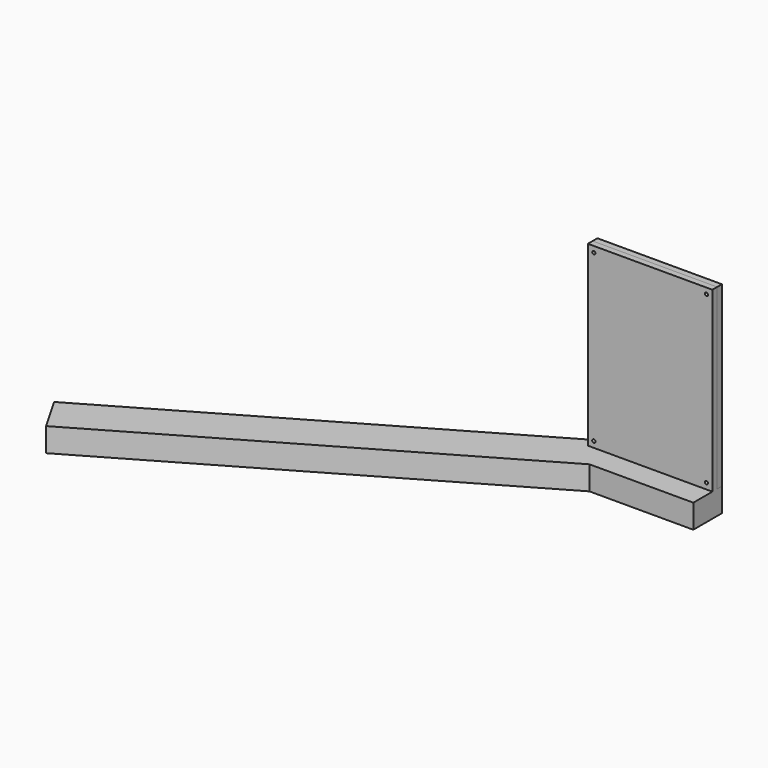
from build123d import *

# Parameters (mm, degrees)
F0_W      = 265.2573054
F0_H      = 378.7020874
F1_DEPTH  = 12.7
F2_DEPTH  = 3.302
F3_W      = 76.2
F3_H      = 50.8
F3_W_2    = 69.85
F3_H_2    = 44.45
F4_DEPTH  = 265.2573054
F6_DEPTH  = 50.8
F7_DEPTH  = 914.4
F8_W      = 265.2573054
F8_H      = 378.7020874
F8_R      = 3.4544
F9_DEPTH  = 12.7
F11_W     = 76.2
F11_H     = 50.8
F12_DEPTH = 3.175


with BuildPart() as f1:
    # F0 (on Front) → F1 (new body)
    with BuildSketch(Plane.XZ):
        with Locations((148.0387565, -1.27e-05)):
            Rectangle(F0_W, F0_H)
        with BuildLine():
            ThreePointArc((24.6557038, -176.6510564), (28.1101038, -173.1966564), (31.5645038, -176.6510564))
            ThreePointArc((31.5645038, -176.6510564), (28.1101038, -180.1054564), (24.6557038, -176.6510564))
        make_face(mode=Mode.SUBTRACT)
        with BuildLine():
            ThreePointArc((264.5130092, -176.6510564), (267.9674092, -173.1966564), (271.4218092, -176.6510564))
            ThreePointArc((271.4218092, -176.6510564), (267.9674092, -180.1054564), (264.5130092, -176.6510564))
        make_face(mode=Mode.SUBTRACT)
        with BuildLine():
            ThreePointArc((24.6557038, 176.651031), (28.1101038, 180.105431), (31.5645038, 176.651031))
            ThreePointArc((31.5645038, 176.651031), (28.1101038, 173.196631), (24.6557038, 176.651031))
        make_face(mode=Mode.SUBTRACT)
        with BuildLine():
            ThreePointArc((264.5130092, 176.651031), (267.9674092, 180.105431), (271.4218092, 176.651031))
            ThreePointArc((271.4218092, 176.651031), (267.9674092, 173.196631), (264.5130092, 176.651031))
        make_face(mode=Mode.SUBTRACT)
    extrude(amount=F1_DEPTH)


with BuildPart() as f1b:
    # F0 (on Front) → F1, piece 2 (new body)
    with BuildSketch(Plane.XZ):
        with BuildLine():
            Line((-259.816473, -139.4988066), (-259.809869, 139.9750058))
            ThreePointArc((-259.8098689962, 139.9750058), (-255.6250403922, 150.0775804789), (-245.522369, 154.2621756))
            Line((-245.522369, 154.2621756), (-50.5753624, 154.2621756))
            ThreePointArc((-50.5753624, 154.2621756), (-40.4724665013, 150.0773559726), (-36.2878624033, 139.9743708))
            Line((-36.2878624, 139.9743708), (-36.2944664, -139.4994416))
            ThreePointArc((-36.2944664038, -139.4994416), (-40.4792950078, -149.6020162789), (-50.5819664, -153.7866114))
            Line((-50.5819664, -153.7866114), (-132.307457, -153.7866114))
            ThreePointArc((-132.307457, -153.7866114), (-134.4627184691, -154.6793499309), (-135.355457, -156.8346114))
            Line((-135.355457, -156.8346114), (-135.355457, -171.7670174))
            Line((-135.355457, -171.7670174), (-135.355457, -187.919233))
            Line((-135.355457, -187.919233), (-135.355457, -189.3510564))
            Line((-135.355457, -189.3510564), (-15.4101038, -189.3510564))
            Line((-15.4101038, -189.3510564), (-15.4101038, 189.351031))
            Line((-15.4101038, 189.351031), (-280.6674092, 189.351031))
            Line((-280.6674092, 189.351031), (-280.6674092, -189.3510564))
            Line((-280.6674092, -189.3510564), (-160.755457, -189.3510564))
            Line((-160.755457, -189.3510564), (-160.755457, -187.919233))
            Line((-160.755457, -187.919233), (-160.755457, -171.7670174))
            Line((-160.755457, -171.7670174), (-160.755457, -156.8346114))
            ThreePointArc((-160.755457, -156.8346114), (-161.6481955309, -154.6793499309), (-163.803457, -153.7866114))
            Line((-163.803457, -153.7866114), (-245.528973, -153.7866114))
            ThreePointArc((-245.528973, -153.7866114), (-255.6318688987, -149.6017917726), (-259.8164729967, -139.4988066))
        make_face()
        with BuildLine():
            ThreePointArc((-271.4218092, -176.6510564), (-267.9674092, -173.1966564), (-264.5130092, -176.6510564))
            ThreePointArc((-264.5130092, -176.6510564), (-267.9674092, -180.1054564), (-271.4218092, -176.6510564))
        make_face(mode=Mode.SUBTRACT)
        with BuildLine():
            ThreePointArc((-31.5645038, -176.6510564), (-28.1101038, -173.1966564), (-24.6557038, -176.6510564))
            ThreePointArc((-24.6557038, -176.6510564), (-28.1101038, -180.1054564), (-31.5645038, -176.6510564))
        make_face(mode=Mode.SUBTRACT)
        with BuildLine():
            ThreePointArc((-271.4218092, 176.651031), (-267.9674092, 180.105431), (-264.5130092, 176.651031))
            ThreePointArc((-264.5130092, 176.651031), (-267.9674092, 173.196631), (-271.4218092, 176.651031))
        make_face(mode=Mode.SUBTRACT)
        with BuildLine():
            ThreePointArc((-31.5645038, 176.651031), (-28.1101038, 180.105431), (-24.6557038, 176.651031))
            ThreePointArc((-24.6557038, 176.651031), (-28.1101038, 173.196631), (-31.5645038, 176.651031))
        make_face(mode=Mode.SUBTRACT)
    extrude(amount=F1_DEPTH)

    # F0 (on Front) → F2 (join)
    with BuildSketch(Plane.XZ):
        with BuildLine():
            ThreePointArc((-245.522369, 154.2621756), (-255.6250403922, 150.0775804789), (-259.8098689962, 139.9750058))
            Line((-259.809869, 139.9750058), (-259.816473, -139.4988066))
            ThreePointArc((-259.8164729967, -139.4988066), (-255.6318688987, -149.6017917726), (-245.528973, -153.7866114))
            Line((-245.528973, -153.7866114), (-163.803457, -153.7866114))
            ThreePointArc((-163.803457, -153.7866114), (-161.6481955309, -154.6793499309), (-160.755457, -156.8346114))
            Line((-160.755457, -156.8346114), (-160.755457, -171.7670174))
            Line((-160.755457, -171.7670174), (-160.755457, -187.919233))
            Line((-160.755457, -187.919233), (-160.755457, -189.3510564))
            Line((-160.755457, -189.3510564), (-135.355457, -189.3510564))
            Line((-135.355457, -189.3510564), (-135.355457, -187.919233))
            Line((-135.355457, -187.919233), (-135.355457, -171.7670174))
            Line((-135.355457, -171.7670174), (-135.355457, -156.8346114))
            ThreePointArc((-135.355457, -156.8346114), (-134.4627184691, -154.6793499309), (-132.307457, -153.7866114))
            Line((-132.307457, -153.7866114), (-50.5819664, -153.7866114))
            ThreePointArc((-50.5819664, -153.7866114), (-40.4792950078, -149.6020162789), (-36.2944664038, -139.4994416))
            Line((-36.2944664, -139.4994416), (-36.2878624, 139.9743708))
            ThreePointArc((-36.2878624033, 139.9743708), (-40.4724665013, 150.0773559726), (-50.5753624, 154.2621756))
            Line((-50.5753624, 154.2621756), (-245.522369, 154.2621756))
        make_face()
        with BuildLine():
            ThreePointArc((-241.6466592, -129.499233), (-243.8917232303, -128.5692970303), (-244.8216592, -126.324233))
            Line((-244.8216592, -126.324233), (-244.8216592, 126.324741))
            ThreePointArc((-244.8216592, 126.324741), (-243.8917232303, 128.5698050303), (-241.6466592, 129.499741))
            Line((-241.6466592, 129.499741), (-54.6371526, 129.499741))
            ThreePointArc((-54.6371526, 129.499741), (-52.3920885697, 128.5698050303), (-51.4621526, 126.324741))
            Line((-51.4621526, 126.324741), (-51.4621526, -126.324233))
            ThreePointArc((-51.4621526, -126.324233), (-52.3920885697, -128.5692970303), (-54.6371526, -129.499233))
            Line((-54.6371526, -129.499233), (-241.6466592, -129.499233))
        make_face(mode=Mode.SUBTRACT)
        with BuildLine():
            ThreePointArc((-31.5645038, 176.651031), (-28.1101038, 173.196631), (-24.6557038, 176.651031))
            ThreePointArc((-24.6557038, 176.651031), (-28.1101038, 180.105431), (-31.5645038, 176.651031))
        make_face()
        with BuildLine():
            ThreePointArc((-31.5645038, -176.6510564), (-28.1101038, -180.1054564), (-24.6557038, -176.6510564))
            ThreePointArc((-24.6557038, -176.6510564), (-28.1101038, -173.1966564), (-31.5645038, -176.6510564))
        make_face()
        with BuildLine():
            ThreePointArc((-271.4218092, -176.6510564), (-267.9674092, -180.1054564), (-264.5130092, -176.6510564))
            ThreePointArc((-264.5130092, -176.6510564), (-267.9674092, -173.1966564), (-271.4218092, -176.6510564))
        make_face()
        with BuildLine():
            ThreePointArc((-271.4218092, 176.651031), (-267.9674092, 173.196631), (-264.5130092, 176.651031))
            ThreePointArc((-264.5130092, 176.651031), (-267.9674092, 180.105431), (-271.4218092, 176.651031))
        make_face()
    extrude(amount=F2_DEPTH)


with BuildPart() as f4:
    # F3 (on face) → F4 (new body, through all)
    with BuildSketch(Plane.YZ.offset(-15.4101038)):
        with Locations((-38.1, -214.7510564)):
            Rectangle(F3_W, F3_H)
        with Locations((-38.1, -214.7510564)):
            Rectangle(F3_W_2, F3_H_2, mode=Mode.SUBTRACT)
    extrude(amount=-F4_DEPTH)

    # F5 (on face) → F6 (cut)
    with BuildSketch(Plane(origin=(0, 0, -240.1510564), x_dir=(1, 0, 0), z_dir=(0, 0, -1))):
        Polygon((-280.6674092001, 76.2), (-280.6674092001, 0), (-236.6733186879, 76.2), align=None)
    extrude(amount=-F6_DEPTH, mode=Mode.SUBTRACT)

    # F7 (add): a face of the model
    f7_faces = [f4.faces().sort_by_distance(p)[0] for p in [
        (-258.670363944, -38.1, -239.1350564),
    ]]
    extrude(f7_faces, amount=F7_DEPTH)

    # F8 (on face) → F9 (join)
    with BuildSketch(Plane.XZ.offset(12.7)):
        with Locations((-148.0387565, -1.27e-05)):
            Rectangle(F8_W, F8_H)
        with Locations((-267.9674092, -176.6510564)):
            Circle(F8_R, mode=Mode.SUBTRACT)
        with Locations((-28.1101038, -176.6510564)):
            Circle(F8_R, mode=Mode.SUBTRACT)
        with Locations((-267.9674092, 176.651031)):
            Circle(F8_R, mode=Mode.SUBTRACT)
        with Locations((-28.1101038, 176.651031)):
            Circle(F8_R, mode=Mode.SUBTRACT)
    extrude(amount=F9_DEPTH)

    # F10: union 

    # F11 (on face) → F12 (join)
    with BuildSketch(Plane.YZ.offset(-15.4101038)):
        with Locations((-38.1, -214.7510564)):
            Rectangle(F11_W, F11_H)
    extrude(amount=-F12_DEPTH)


solid = Compound([f1b.part, f4.part])
